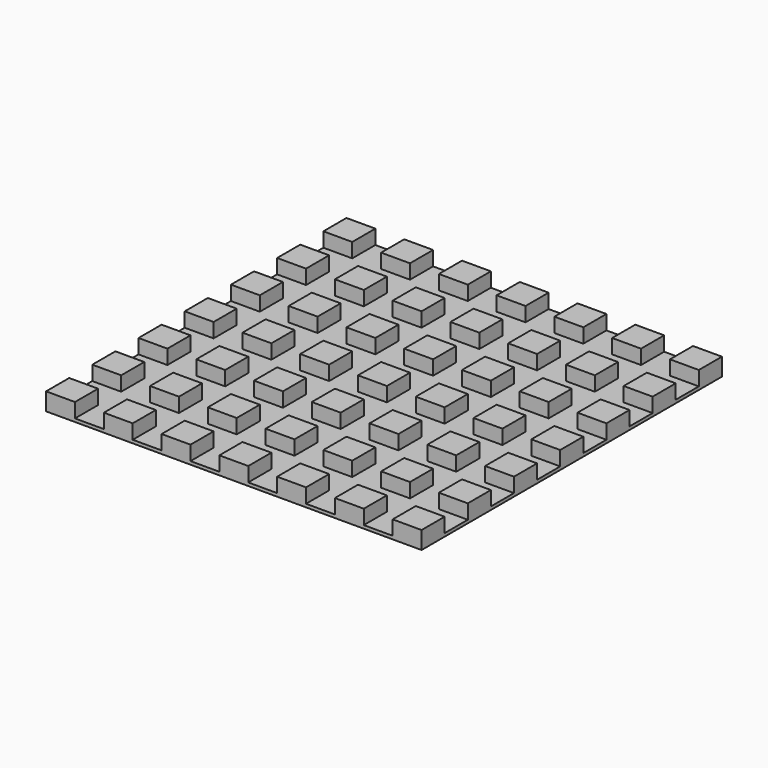
from build123d import *

# Parameters (mm, degrees)
F0_W         = 130
F0_H         = 130
F1_DEPTH     = 1.1
F2_W         = 10
F2_H         = 10
F3_DEPTH     = 5
F4_TEXT_SIZE = 16.7890870934
F5_DEPTH     = 0.5


# Not quite as in the source:
# - Text() gives the source's letters only with a copy of the font that has no kerning and outlines rounded to 1/6400 em; it was checked with that copy


with BuildPart() as f1:
    # F0 (on Top) → F1 (new body)
    with BuildSketch(Plane.XY):
        with Locations((65, 65)):
            Rectangle(F0_W, F0_H)
    extrude(amount=F1_DEPTH)

    # F2 (on face) → F3 (join)
    with BuildSketch(Plane.XY.offset(1.1)):
        with Locations((5, 5)):
            Rectangle(F2_W, F2_H)
        with Locations((5, 25)):
            Rectangle(F2_W, F2_H)
        with Locations((5, 45)):
            Rectangle(F2_W, F2_H)
        with Locations((5, 65)):
            Rectangle(F2_W, F2_H)
        with Locations((5, 85)):
            Rectangle(F2_W, F2_H)
        with Locations((5, 105)):
            Rectangle(F2_W, F2_H)
        with Locations((25, 5)):
            Rectangle(F2_W, F2_H)
        with Locations((25, 25)):
            Rectangle(F2_W, F2_H)
        with Locations((25, 45)):
            Rectangle(F2_W, F2_H)
        with Locations((25, 65)):
            Rectangle(F2_W, F2_H)
        with Locations((25, 85)):
            Rectangle(F2_W, F2_H)
        with Locations((25, 105)):
            Rectangle(F2_W, F2_H)
        with Locations((45, 5)):
            Rectangle(F2_W, F2_H)
        with Locations((45, 25)):
            Rectangle(F2_W, F2_H)
        with Locations((45, 45)):
            Rectangle(F2_W, F2_H)
        with Locations((45, 65)):
            Rectangle(F2_W, F2_H)
        with Locations((45, 85)):
            Rectangle(F2_W, F2_H)
        with Locations((45, 105)):
            Rectangle(F2_W, F2_H)
        with Locations((65, 5)):
            Rectangle(F2_W, F2_H)
        with Locations((65, 25)):
            Rectangle(F2_W, F2_H)
        with Locations((65, 45)):
            Rectangle(F2_W, F2_H)
        with Locations((65, 65)):
            Rectangle(F2_W, F2_H)
        with Locations((65, 85)):
            Rectangle(F2_W, F2_H)
        with Locations((65, 105)):
            Rectangle(F2_W, F2_H)
        with Locations((85, 5)):
            Rectangle(F2_W, F2_H)
        with Locations((85, 25)):
            Rectangle(F2_W, F2_H)
        with Locations((85, 45)):
            Rectangle(F2_W, F2_H)
        with Locations((85, 65)):
            Rectangle(F2_W, F2_H)
        with Locations((85, 85)):
            Rectangle(F2_W, F2_H)
        with Locations((85, 105)):
            Rectangle(F2_W, F2_H)
        with Locations((105, 5)):
            Rectangle(F2_W, F2_H)
        with Locations((105, 25)):
            Rectangle(F2_W, F2_H)
        with Locations((105, 45)):
            Rectangle(F2_W, F2_H)
        with Locations((105, 65)):
            Rectangle(F2_W, F2_H)
        with Locations((105, 85)):
            Rectangle(F2_W, F2_H)
        with Locations((105, 105)):
            Rectangle(F2_W, F2_H)
        with Locations((5, 125)):
            Rectangle(F2_W, F2_H)
        with Locations((25, 125)):
            Rectangle(F2_W, F2_H)
        with Locations((45, 125)):
            Rectangle(F2_W, F2_H)
        with Locations((65, 125)):
            Rectangle(F2_W, F2_H)
        with Locations((85, 125)):
            Rectangle(F2_W, F2_H)
        with Locations((105, 125)):
            Rectangle(F2_W, F2_H)
        with Locations((125, 5)):
            Rectangle(F2_W, F2_H)
        with Locations((125, 25)):
            Rectangle(F2_W, F2_H)
        with Locations((125, 45)):
            Rectangle(F2_W, F2_H)
        with Locations((125, 65)):
            Rectangle(F2_W, F2_H)
        with Locations((125, 85)):
            Rectangle(F2_W, F2_H)
        with Locations((125, 105)):
            Rectangle(F2_W, F2_H)
        with Locations((125, 125)):
            Rectangle(F2_W, F2_H)
    extrude(amount=F3_DEPTH)

    # F4 (on face) → F5 (cut)
    with BuildSketch(Plane(origin=(0, 0, 0), x_dir=(1, 0, 0), z_dir=(0, 0, -1))):
        with Locations((60, -125)):
            Text('Z', F4_TEXT_SIZE, font='Open Sans', text_align=(TextAlign.LEFT, TextAlign.BOTTOM))
    extrude(amount=-F5_DEPTH, mode=Mode.SUBTRACT)


solid = f1.part
